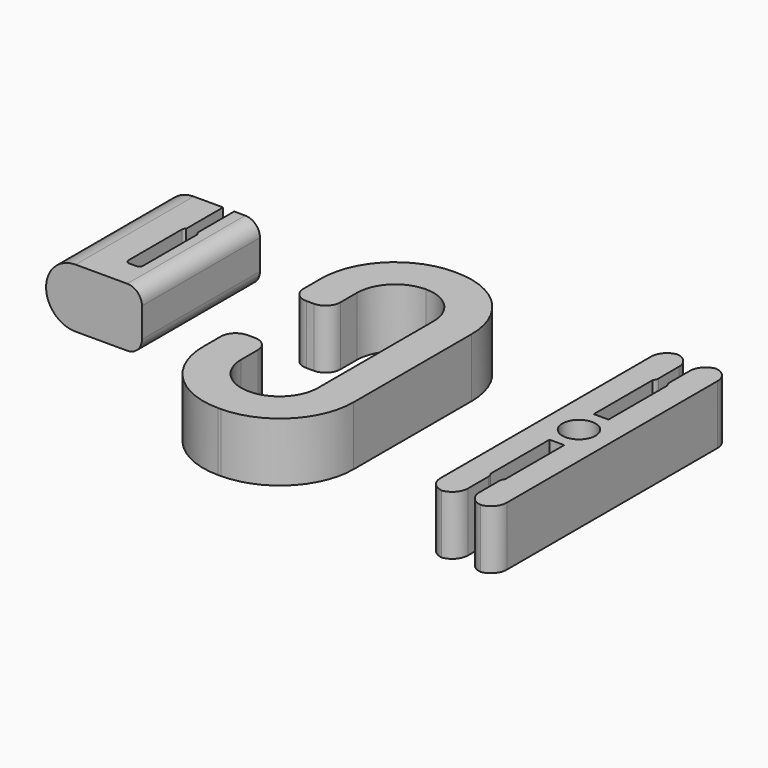
from build123d import *

# Parameters (mm, degrees)
F1_DEPTH     = 8
F2_R         = 5.19999
F3_R         = 10
F6_DEPTH     = 8
F7_R         = 2.25
F8_DEPTH     = 8
F9_T1_DEPTH  = 18.75
F10_T1_DEPTH = 11.3071891388
F12_DEPTH    = 8
F13_R        = 2.25
F14_DEPTH    = 15
F15_R        = 3.99999
F16_T1_DEPTH = 8
F17_R        = 2
F17_2_R      = 2


# Not quite as in the source:
# - a fillet or chamfer that OpenCascade refuses, or shapes differently, is made with other operations: its cross-section is extruded or revolved along the edge and cut away or added
# - a fillet or chamfer is up to 0.001 mm smaller than in the source, because OpenCascade refuses the exact size
# - a feature of the source that left no trace in its solid (it failed there, or was rolled back) is left out


with BuildPart() as f1:
    # F0 (on Top) → F1 (new body)
    with BuildSketch(Plane.XY):
        Polygon((-5.2, 15), (5.2, 15), (5.2, -15), (-5.2, -15), (-5.2, -5), (-10.2, -5), (-10.2, -20), (10.2, -20), (10.2, 20), (-10.2, 20), (-10.2, 5), (-5.2, 5), align=None)
    extrude(amount=F1_DEPTH)

    # F2 (radius 5.2 in the source; OpenCascade refuses exactly that, so slightly less here)
    f2_edges = [f1.edges().sort_by_distance(p)[0] for p in [
        (-5.2, 15, 4),
        (5.2, 15, 4),
        (-5.2, -15, 4),
        (5.2, -15, 4),
    ]]
    fillet(f2_edges, radius=F2_R)

    # F3
    f3_edges = [f1.edges().sort_by_distance(p)[0] for p in [
        (-10.2, 20, 4),
        (10.2, 20, 4),
        (10.2, -20, 4),
        (-10.2, -20, 4),
    ]]
    fillet(f3_edges, radius=F3_R)

    # F17#2
    f17_2_edges = [f1.edges().sort_by_distance(p)[0] for p in [
        (-10.2, 5, 4),
        (-5.2, 5, 4),
        (-10.2, -5, 4),
        (-5.2, -5, 4),
    ]]
    fillet(f17_2_edges, radius=F17_2_R)


with BuildPart() as f6:
    # F5 (on Top) → F6 (new body)
    with BuildSketch(Plane.XY):
        Polygon((32, 20), (31.75, 20), (28.25, 20), (28.25, -20), (31.75, -20), (32, -20), (32, -13.75), (31.75, -13.75), (31.75, -3.75), (33.75, -3.75), (33.75, -13.75), (33.5, -13.75), (33.5, -20), (33.75, -20), (37.25, -20), (37.25, 20), (33.75, 20), (33.5, 20), (33.5, 13.75), (33.75, 13.75), (33.75, 3.75), (31.75, 3.75), (31.75, 13.75), (32, 13.75), align=None)
    extrude(amount=F6_DEPTH)

    # F7 (on face) → F8 (cut, through all)
    with BuildSketch(Plane(origin=(0, 0, 0), x_dir=(1, 0, 0), z_dir=(0, 0, -1))):
        with Locations((32.75, 0)):
            Circle(F7_R)
    extrude(amount=-F8_DEPTH, mode=Mode.SUBTRACT)

    # F9: fillet of radius 2.15 on 8 edges, made by hand

    # F9_s2 → F9_t1 (cut)
    with BuildSketch(Plane.XY.offset(-5.375)):
        with BuildLine():
            ThreePointArc((28.25, -17.85), (28.8797204204, -19.3702795796), (30.4, -20))
            Line((30.4, -20), (28.25, -20))
            Line((28.25, -20), (28.25, -17.85))
        make_face()
        with BuildLine():
            ThreePointArc((29.85, -20), (31.3702795796, -19.3702795796), (32, -17.85))
            Line((32, -17.85), (32, -20))
            Line((32, -20), (29.85, -20))
        make_face()
        with BuildLine():
            ThreePointArc((37.25, -17.85), (36.6202795796, -19.3702795796), (35.1, -20))
            Line((35.1, -20), (37.25, -20))
            Line((37.25, -20), (37.25, -17.85))
        make_face()
        with BuildLine():
            ThreePointArc((33.5, -17.85), (34.1297204204, -19.3702795796), (35.65, -20))
            Line((35.65, -20), (33.5, -20))
            Line((33.5, -20), (33.5, -17.85))
        make_face()
        with BuildLine():
            ThreePointArc((35.1, 20), (36.6202795796, 19.3702795796), (37.25, 17.85))
            Line((37.25, 17.85), (37.25, 20))
            Line((37.25, 20), (35.1, 20))
        make_face()
        with BuildLine():
            ThreePointArc((33.5, 17.85), (34.1297204204, 19.3702795796), (35.65, 20))
            Line((35.65, 20), (33.5, 20))
            Line((33.5, 20), (33.5, 17.85))
        make_face()
        with BuildLine():
            ThreePointArc((29.85, 20), (31.3702795796, 19.3702795796), (32, 17.85))
            Line((32, 17.85), (32, 20))
            Line((32, 20), (29.85, 20))
        make_face()
        with BuildLine():
            ThreePointArc((30.4, 20), (28.8797204204, 19.3702795796), (28.25, 17.85))
            Line((28.25, 17.85), (28.25, 20))
            Line((28.25, 20), (30.4, 20))
        make_face()
    extrude(amount=F9_T1_DEPTH, mode=Mode.SUBTRACT)

    # F10: fillet of radius 1 on 4 edges, made by hand

    # F10_s2 → F10_t1 (cut)
    with BuildSketch(Plane.XY.offset(-1.6535945694)):
        with BuildLine():
            ThreePointArc((33.5, -14.4114378278), (33.5645856533, -14.0578844372), (33.75, -13.75))
            Line((33.75, -13.75), (33.5, -13.75))
            Line((33.5, -13.75), (33.5, -14.4114378278))
        make_face()
        with BuildLine():
            ThreePointArc((31.75, -13.75), (31.9354143467, -14.0578844372), (32, -14.4114378278))
            Line((32, -14.4114378278), (32, -13.75))
            Line((32, -13.75), (31.75, -13.75))
        make_face()
        with BuildLine():
            ThreePointArc((32, 14.4114378278), (31.9354143467, 14.0578844372), (31.75, 13.75))
            Line((31.75, 13.75), (32, 13.75))
            Line((32, 13.75), (32, 14.4114378278))
        make_face()
        with BuildLine():
            ThreePointArc((33.75, 13.75), (33.5645856533, 14.0578844372), (33.5, 14.4114378278))
            Line((33.5, 14.4114378278), (33.5, 13.75))
            Line((33.5, 13.75), (33.75, 13.75))
        make_face()
    extrude(amount=F10_T1_DEPTH, mode=Mode.SUBTRACT)


with BuildPart() as f12:
    # F11 (on Top) → F12 (new body)
    with BuildSketch(Plane.XY):
        Polygon((-23.5, -3.75), (-23.5, 16.25), (-27, 16.25), (-27, 10), (-26.75, 10), (-26.75, 0), (-28.75, 0), (-28.75, 10), (-28.5, 10), (-28.5, 16.25), (-36.5, 16.25), (-36.5, -3.75), align=None)
    extrude(amount=F12_DEPTH)

    # F13 (on face) → F14 (cut)
    with BuildSketch(Plane(origin=(0, 16.25, 0), x_dir=(-1, 0, 0), z_dir=(0, 1, 0))):
        with Locations((32.625, 4)):
            Circle(F13_R)
    extrude(amount=-F14_DEPTH, mode=Mode.SUBTRACT)

    # F15 (radius 4 in the source; OpenCascade refuses exactly that, so slightly less here)
    f15_edges = [f12.edges().sort_by_distance(p)[0] for p in [
        (-36.5, 6.25, 8),
        (-36.5, 6.25, 0),
    ]]
    fillet(f15_edges, radius=F15_R)

    # F16: fillet of radius 0.5 on 4 edges, made by hand

    # F16_s2 → F16_t1 (join)
    with BuildSketch(Plane.XY):
        with BuildLine():
            ThreePointArc((-26.75, 9.5669872981), (-26.8169872981, 9.8169872981), (-27, 10))
            Line((-27, 10), (-26.75, 10))
            Line((-26.75, 10), (-26.75, 9.5669872981))
        make_face()
        with BuildLine():
            ThreePointArc((-28.5, 10), (-28.6830127019, 9.8169872981), (-28.75, 9.5669872981))
            Line((-28.75, 9.5669872981), (-28.75, 10))
            Line((-28.75, 10), (-28.5, 10))
        make_face()
        with BuildLine():
            ThreePointArc((-28.75, 0.5), (-28.6035533906, 0.1464466094), (-28.25, 0))
            Line((-28.25, 0), (-28.75, 0))
            Line((-28.75, 0), (-28.75, 0.5))
        make_face()
        with BuildLine():
            ThreePointArc((-27.25, 0), (-26.8964466094, 0.1464466094), (-26.75, 0.5))
            Line((-26.75, 0.5), (-26.75, 0))
            Line((-26.75, 0), (-27.25, 0))
        make_face()
    extrude(amount=F16_T1_DEPTH)

    # F17
    f17_edges = [f12.edges().sort_by_distance(p)[0] for p in [
        (-23.5, 6.25, 8),
        (-23.5, 6.25, 0),
    ]]
    fillet(f17_edges, radius=F17_R)


solid = Compound([f1.part, f6.part, f12.part])
